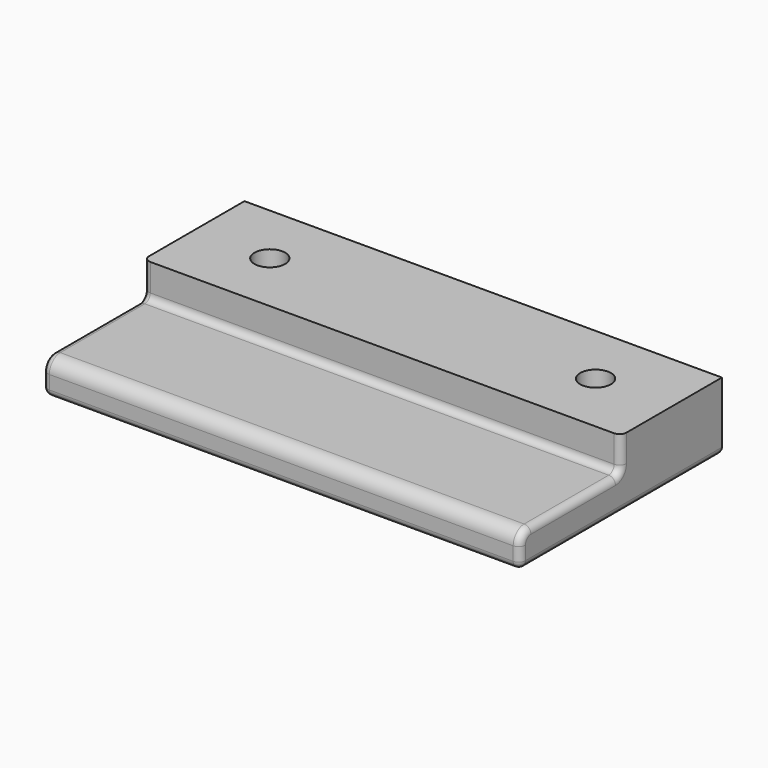
from build123d import *

# Parameters (mm, degrees)
F0_W           = 70
F0_H           = 18.5
F1_DEPTH       = 10
F2_DEPTH       = 5
F3_R           = 2
F4_R           = 1
F5_D           = 4.5
F5_CSINK_D     = 7
F5_CSINK_ANGLE = 90


with BuildPart() as f1:
    # F0 (on Top) → F1 (new body)
    with BuildSketch(Plane.XY):
        with Locations((15.0051557424, 0)):
            Rectangle(F0_W, F0_H)
    extrude(amount=F1_DEPTH)

    # F0 (on Top) → F2 (join)
    with BuildSketch(Plane.XY):
        with Locations((15.0051557424, -18.5)):
            Rectangle(F0_W, F0_H)
    extrude(amount=F2_DEPTH)

    # F3
    f3_edges = [f1.edges().sort_by_distance(p)[0] for p in [
        (15.005156, -27.75, 5),
    ]]
    fillet(f3_edges, radius=F3_R)

    # F4
    f4_edges = [f1.edges().sort_by_distance(p)[0] for p in [
        (50.005156, -17.5, 5),
        (-19.994844, -17.5, 5),
        (50.005156, -9.25, 0),
        (15.005156, -27.75, 0),
        (-19.994844, -9.25, 0),
        (15.005156, 9.25, 0),
        (15.005156, -9.25, 5),
        (-19.994844, -27.164214, 4.414214),
        (-19.994844, -9.25, 7.5),
        (50.005156, -27.164214, 4.414214),
        (50.005156, -9.25, 7.5),
    ]]
    fillet(f4_edges, radius=F4_R)

    # F5 (through all)
    with Locations(Plane(origin=(0, 0, 0), x_dir=(1, 0, 0), z_dir=(0, 0, -1))):
        with Locations((-8.8698442576, 0), (38.8801557424, 0)):
            CounterSinkHole(F5_D / 2, F5_CSINK_D / 2, counter_sink_angle=F5_CSINK_ANGLE)


solid = f1.part
